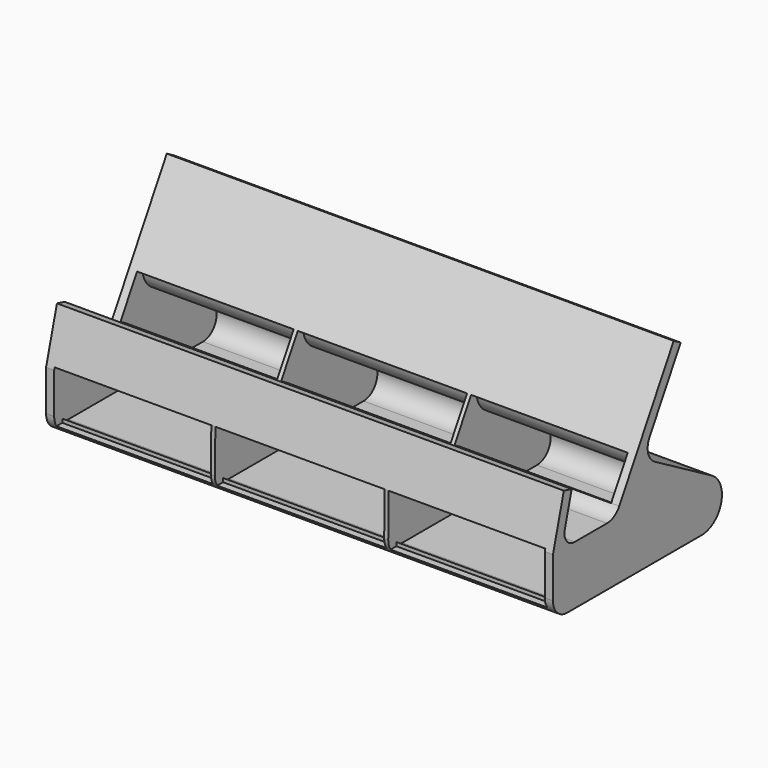
from build123d import *

# Parameters (mm, degrees)
F1_DEPTH    = 100
F2_R        = 7
F3_T1_DEPTH = 386.6025403784
F4_T        = -3.2
F5_W        = 193.6
F5_H        = 20.7961232061
F6_DEPTH    = 4
F9_DEPTH    = 1.6
F10_W       = 61.8
F10_H       = 16.3858774256
F10_W_2     = 66.8
F11_DEPTH   = 3.25


# Not quite as in the source:
# - a fillet or chamfer that OpenCascade refuses, or shapes differently, is made with other operations: its cross-section is extruded or revolved along the edge and cut away or added
# - a pattern or mirror of a feature is missing from the dataset's text; its kind, count and spacing are read off the source's solid


with BuildPart() as f1:
    # F0 (on Right) → F1 (new body, symmetric)
    with BuildSketch(Plane.YZ):
        with BuildLine():
            ThreePointArc((-42.8978583449, -31.6602540378), (-46.8646250463, -29.7040611829), (-47.7274874763, -25.3661588123))
            Line((-47.7274874763, -25.3661588123), (-44.3324027769, -12.6955302183))
            Line((-44.3324027769, -12.6955302183), (-48.1961060821, -11.6602540378))
            Line((-48.1961060821, -11.6602540378), (-53.5550899307, -31.6602540378))
            Line((-53.5550899307, -31.6602540378), (-53.5550899307, -54.7542648054))
            Line((-53.5550899307, -54.7542648054), (57.1021416551, -54.7542648054))
            Line((57.1021416551, -54.7542648054), (-9.4337567297, -16.3397459622))
            Line((-9.4337567297, -16.3397459622), (9.4337567297, 16.3397459622))
            Line((9.4337567297, 16.3397459622), (5.9696551146, 18.3397459622))
            Line((5.9696551146, 18.3397459622), (-22.8978583449, -31.6602540378))
            Line((-22.8978583449, -31.6602540378), (-42.8978583449, -31.6602540378))
        make_face()
    extrude(amount=F1_DEPTH, both=True)

    # F2
    f2_edges = [f1.edges().sort_by_distance(p)[0] for p in [
        (0, -53.55509, -54.754265),
        (0, -9.433757, -16.339746),
        (0, -22.897858, -31.660254),
    ]]
    fillet(f2_edges, radius=F2_R)

    # F3: fillet of radius 10 on 1 edges, made by hand

    # F3_s2 → F3_t1 (cut)
    with BuildSketch(Plane.YZ.offset(-193.3012701892)):
        with BuildLine():
            ThreePointArc((24.7816335794, -36.0940107676), (29.4408918423, -47.3424552565), (19.7816335794, -54.7542648054))
            Line((19.7816335794, -54.7542648054), (57.1021416551, -54.7542648054))
            Line((57.1021416551, -54.7542648054), (24.7816335794, -36.0940107676))
        make_face()
    extrude(amount=F3_T1_DEPTH, mode=Mode.SUBTRACT)

    # F4 (hollow: no face is removed)
    offset(amount=F4_T, mode=Mode.SUBTRACT)

    # F5 (on face) → F6 (cut)
    with BuildSketch(Plane.XZ.offset(53.5550899307)):
        with Locations((0, -41.1562032024)):
            Rectangle(F5_W, F5_H)
    extrude(amount=-F6_DEPTH, mode=Mode.SUBTRACT)

    # F8 (on offset) → F9 (join)
    with BuildSketch(Plane.YZ.offset(35)):
        with BuildLine():
            Line((-49.5550899307, -31.4478701056), (-49.5550899307, -30.7581415993))
            Line((-49.5550899307, -30.7581415993), (-53.3133696313, -30.7581415993))
            Line((-53.3133696313, -30.7581415993), (-53.5550899307, -47.7542648054))
            ThreePointArc((-53.5550899307, -47.7542648054), (-53.2689348678, -49.735245916), (-52.4338653134, -51.5542648054))
            Line((-52.4338653134, -51.5542648054), (-46.5550899307, -51.5542648054))
            Line((-46.5550899307, -51.5542648054), (19.7816335794, -51.5542648054))
            ThreePointArc((19.7816335794, -51.5542648054), (26.3499291982, -46.5142343121), (23.1816335794, -38.8652920597))
            Line((23.1816335794, -38.8652920597), (-4.9715789032, -22.6110272543))
            ThreePointArc((-4.9715789032, -22.6110272543), (-8.2208411642, -19.6367335794), (-9.9129123978, -15.569667924))
            Line((-9.9129123978, -15.569667924), (-18.1058511106, -29.7602540378))
            ThreePointArc((-18.1058511106, -29.7602540378), (-21.8393102292, -33.4937131564), (-26.9393102292, -34.8602540378))
            Line((-26.9393102292, -34.8602540378), (-42.8978583449, -34.8602540378))
            ThreePointArc((-42.8978583449, -34.8602540378), (-46.6382826687, -33.9574607553), (-49.5550899307, -31.4478701056))
        make_face()
    f9 = extrude(amount=-F9_DEPTH)

    # F9_copies: F9 across plane
    add(f9.mirror(Plane(origin=(0, 0, 0), x_dir=(0, 0, -1), z_dir=(-1, 0, 0))))

    # F10 (on face) → F11 (cut)
    with BuildSketch(Plane(origin=(0, -3.4641016151, 2), x_dir=(1, 0, 0), z_dir=(0, -0.8660254038, 0.5))):
        with Locations((-65.9, -26.6331228623)):
            Rectangle(F10_W, F10_H)
        with Locations((0, -26.6331228623)):
            Rectangle(F10_W_2, F10_H)
        with Locations((65.9, -26.6331228623)):
            Rectangle(F10_W, F10_H)
    extrude(amount=-F11_DEPTH, mode=Mode.SUBTRACT)


solid = f1.part
